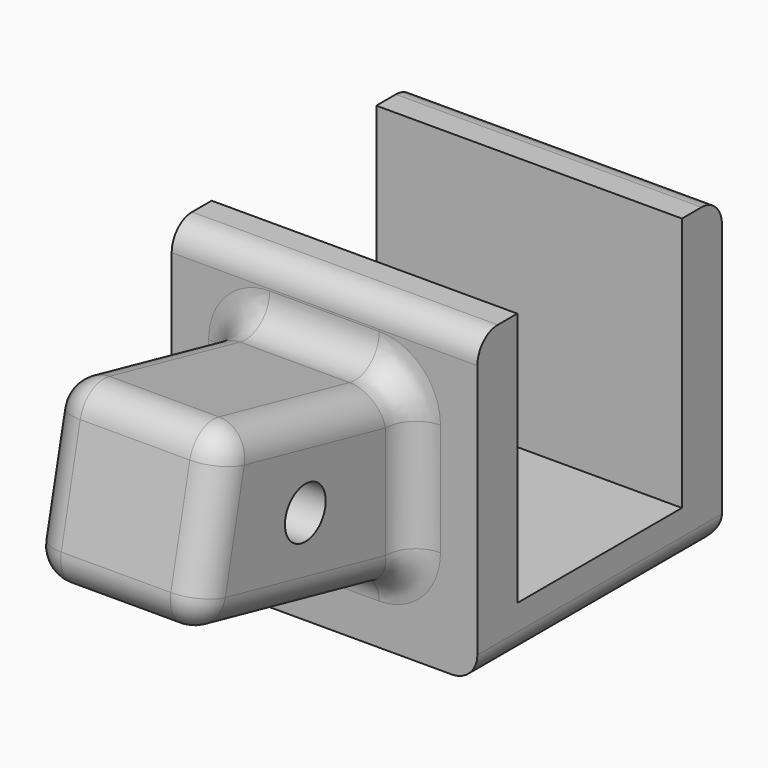
from build123d import *

# Parameters (mm, degrees)
F0_W      = 30
F0_H      = 30
F1_DEPTH  = 5
F2_W      = 30
F2_H      = 4.9
F3_DEPTH  = 25
F6_W      = 16.75
F6_H      = 16.75
F7_DEPTH  = 25
F7_FACE_W = 16.75
F7_FACE_H = 8.375
F9_R      = 3
F10_R     = 2.5
F12_R     = 2.5
F13_DEPTH = 16.75


# Not quite as in the source:
# - two fillets or chamfers of one size are made in one step
# - a feature names something its author has since deleted; it is built from what else it names


with BuildPart() as f1:
    # F0 (on Top) → F1 (new body)
    with BuildSketch(Plane.XY):
        with Locations((15, 15)):
            Rectangle(F0_W, F0_H)
    extrude(amount=F1_DEPTH)

    # F2 (on face) → F3 (join)
    with BuildSketch(Plane.XY.offset(5)):
        with Locations((15, 27.55)):
            Rectangle(F2_W, F2_H)
        with Locations((15, 2.45)):
            Rectangle(F2_W, F2_H)
    extrude(amount=F3_DEPTH)

    # F6 (on line) → F7 (join)
    with BuildSketch(Plane(origin=(0, -3.1696369631, 0.7026915972), x_dir=(1, 0, 0), z_dir=(0, -0.9762960071, 0.2164396139))):
        with Locations((15, 14.6444401068)):
            Rectangle(F6_W, F6_H)
    extrude(amount=F7_DEPTH)

    # F7_face (on face) → F8 (join, up to the next surface of F1)
    with BuildSketch(Plane(origin=(15, -0.9063408834, 10.9117604702), x_dir=(1, 0, 0), z_dir=(0, 0.9762960071, -0.2164396139))):
        Rectangle(F7_FACE_W, F7_FACE_H)
    extrude(until=Until.NEXT)

    # F9
    f9_edges = [f1.edges().sort_by_distance(p)[0] for p in [
        (6.625, -24.4074, 20.41099),
        (23.375, 0, 15),
        (23.375, -13.110041, 9.328085),
        (23.375, -24.4074, 20.41099),
        (23.375, -11.297359, 26.082905),
        (15, 0, 23.578341),
        (6.625, 0, 15),
        (15, 0, 6.421659),
        (6.625, -13.110041, 9.328085),
        (15, -26.220082, 12.234511),
        (15, -22.594718, 28.587469),
        (6.625, -11.297359, 26.082905),
    ]]
    fillet(f9_edges, radius=F9_R)

    # F10
    f10_edges = [f1.edges().sort_by_distance(p)[0] for p in [
        (15, 30, 30),
        (15, 0, 30),
        (15, 30, 0),
        (30, 15, 0),
        (0, 15, 0),
    ]]
    fillet(f10_edges, radius=F10_R)

    # F12 (on face) → F13 (cut, through all)
    with BuildSketch(Plane.YZ.offset(23.375)):
        with Locations((-12.8209375408, 17.8423334229)):
            Circle(F12_R)
    extrude(amount=-F13_DEPTH, mode=Mode.SUBTRACT)


solid = f1.part
